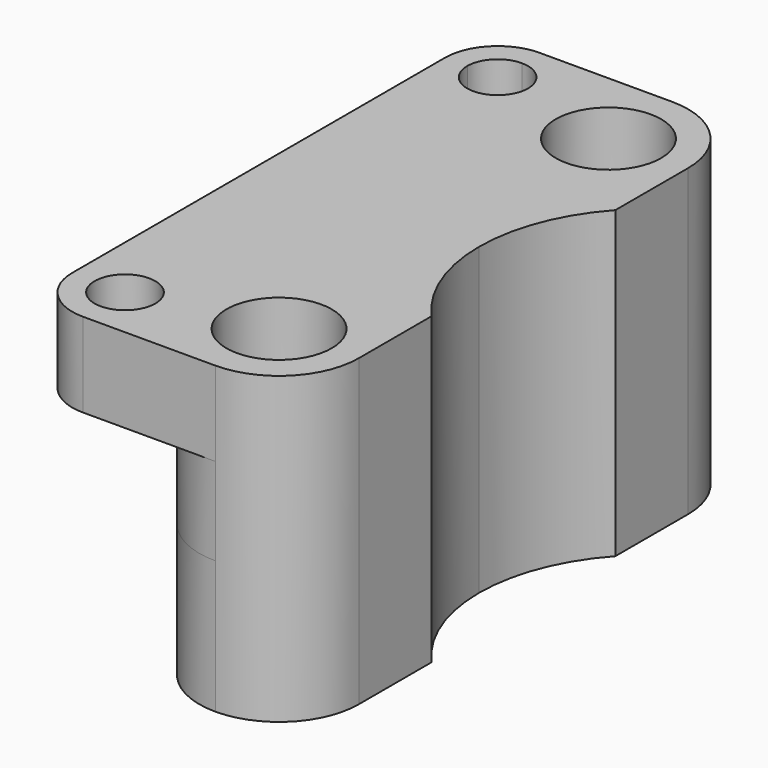
from build123d import *

# Parameters (mm, degrees)
F1_DEPTH = 10
F2_R     = 3.96875
F3_DEPTH = 12.93749
F4_R     = 6.002975
F5_R     = 3.96875
F7_DEPTH = 22.93749
F8_DEPTH = 6.58749


# Not quite as in the source:
# - a fillet or chamfer is up to 0.001 mm smaller than in the source, because OpenCascade refuses the exact size


with BuildPart() as f1:
    # F0 (on Top) → F1 (new body)
    with BuildSketch(Plane.XY):
        Polygon((6.0029852, 0), (0, 0), (0, -43.0059592), (6.0029852, -43.0059592), (12.0059704, -43.0059592), (12.0059704, 0), align=None)
        with BuildLine():
            ThreePointArc((7.5029852, -37.002974), (7.0636453718, -38.0636341718), (6.0029852, -38.502974))
            ThreePointArc((6.0029852, -38.502974), (4.5029852, -37.002974), (6.0029852, -35.502974))
            ThreePointArc((6.0029852, -35.502974), (7.0636453718, -35.9423138282), (7.5029852, -37.002974))
        make_face(mode=Mode.SUBTRACT)
        with BuildLine():
            ThreePointArc((6.0029852, -7.5029852), (4.5029852, -6.0029852), (6.0029852, -4.5029852))
            ThreePointArc((6.0029852, -4.5029852), (7.0636453718, -4.9423250282), (7.5029852, -6.0029852))
            ThreePointArc((7.5029852, -6.0029852), (7.0636453718, -7.0636453718), (6.0029852, -7.5029852))
        make_face(mode=Mode.SUBTRACT)
    extrude(amount=F1_DEPTH)

    # F2 (on face) → F3 (join)
    with BuildSketch(Plane.XY.offset(10)):
        with BuildLine():
            Line((12.0059704, -43.0059592), (12.0059704, 0))
            Line((12.0059704, 0), (-3.96875, 0))
            Line((-3.96875, 0), (-3.96875, -1.68275))
            ThreePointArc((-3.96875, -1.68275), (-2.3523038982, -2.3523038982), (-1.68275, -3.96875))
            ThreePointArc((-1.68275, -3.96875), (-3.96875, -6.25475), (-6.25475, -3.96875))
            Line((-6.25475, -3.96875), (-7.9375, -3.96875))
            Line((-7.9375, -3.96875), (-7.9375, -43.0059592))
            Line((-7.9375, -43.0059592), (-3.96875, -43.0059592))
            Line((-3.96875, -43.0059592), (12.0059704, -43.0059592))
        make_face()
        with BuildLine():
            ThreePointArc((-1.68275, -39.0372092), (-2.3523038982, -40.6536553018), (-3.96875, -41.3232092))
            ThreePointArc((-3.96875, -41.3232092), (-5.5851961018, -37.4207630982), (-1.68275, -39.0372092))
        make_face(mode=Mode.SUBTRACT)
        with Locations((6.0029852, -37.002974)):
            Circle(F2_R, mode=Mode.SUBTRACT)
        with Locations((6.0029852, -6.0029852)):
            Circle(F2_R, mode=Mode.SUBTRACT)
        with BuildLine():
            Line((-3.96875, -1.68275), (-3.96875, 0))
            Line((-3.96875, 0), (-7.9375, 0))
            Line((-7.9375, 0), (-7.9375, -3.96875))
            Line((-7.9375, -3.96875), (-6.25475, -3.96875))
            ThreePointArc((-6.25475, -3.96875), (-5.5851961018, -2.3523038982), (-3.96875, -1.68275))
        make_face()
    extrude(amount=F3_DEPTH)

    # F4 (radius 6.0029852 in the source; OpenCascade refuses exactly that, so slightly less here)
    f4_edges = [f1.edges().sort_by_distance(p)[0] for p in [
        (12.00597, 0, 11.468745),
        (0, 0, 5),
        (0, -43.005959, 5),
        (12.00597, -43.005959, 11.468745),
    ]]
    fillet(f4_edges, radius=F4_R)

    # F5
    f5_edges = [f1.edges().sort_by_distance(p)[0] for p in [
        (-7.9375, -43.005959, 16.468745),
        (-7.9375, 0, 16.468745),
    ]]
    fillet(f5_edges, radius=F5_R)

    # F6 (on face) → F7 (cut, through all)
    with BuildSketch(Plane(origin=(0, 0, 0), x_dir=(1, 0, 0), z_dir=(0, 0, -1))):
        with BuildLine():
            ThreePointArc((12.0059704, 30.145029001), (9.5274974569, 26.1361174223), (8.6624922, 21.5029796))
            Line((8.6624922, 21.5029796), (12.0059704, 21.5029796))
            Line((12.0059704, 21.5029796), (12.0059704, 30.145029001))
        make_face()
        with BuildLine():
            Line((12.0059704, 21.5029796), (8.6624922, 21.5029796))
            ThreePointArc((8.6624922, 21.5029796), (9.5274974569, 16.8698417777), (12.0059704, 12.860930199))
            Line((12.0059704, 12.860930199), (12.0059704, 21.5029796))
        make_face()
    extrude(amount=-F7_DEPTH, mode=Mode.SUBTRACT)

    # F8 (cut): a face of the model
    f8_faces = [f1.faces().sort_by_distance(p)[0] for p in [
        (-3.6441940758, -21.5029796, 10),
    ]]
    extrude(f8_faces, amount=-F8_DEPTH, mode=Mode.SUBTRACT)


solid = f1.part
